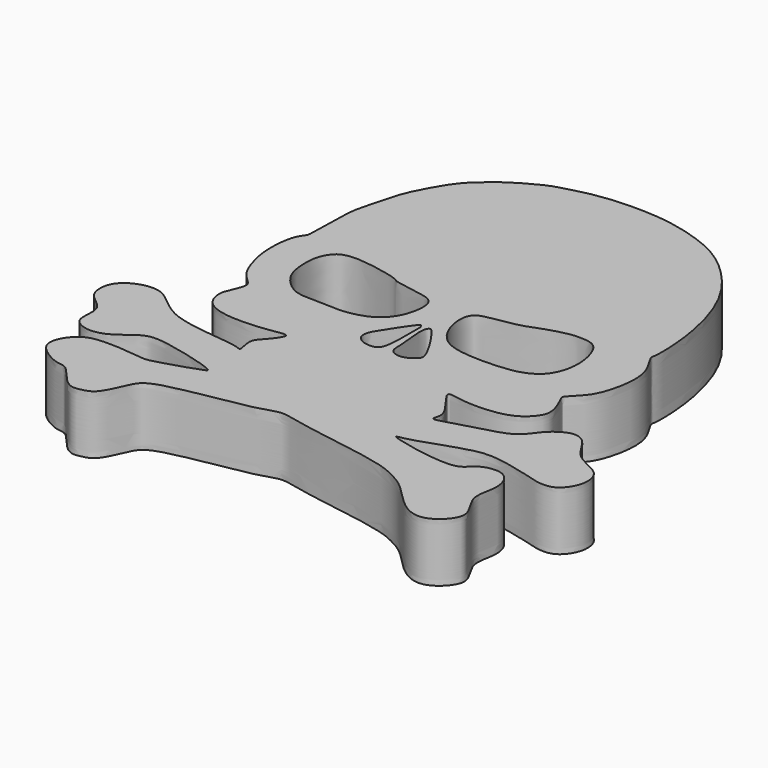
from build123d import *

# Parameters (mm, degrees)
F2_DEPTH = 5


# Not quite as in the source:
# - the program builds the solid bodies; features that only make, move or delete a surface that nothing else refers to are left out


with BuildPart() as f2:
    # F0 (on Top) → F2 (new body)
    with BuildSketch(Plane.XY):
        with BuildLine():
            add(Edge.make_bspline(
                [(0, 29.1948150843), (-0.455700376, 29.1905925458), (-1.1567215924, 29.1618461529), (-3.1403467697, 28.9760038822), (-5.3502695562, 28.3451092019), (-6.2987855508, 28.08405076), (-8.7371541954, 26.7472490664), (-9.9789020308, 25.6205862946), (-11.1795496875, 24.6292942159), (-12.7218376486, 21.8252572969), (-13.1883939862, 20.579718657), (-13.7634070057, 18.2333096853), (-14.1852851071, 16.8622027364), (-14.1170047877, 12.8287797099), (-14.2482133356, 12.4533380127), (-14.8390084605, 11.7676672429), (-15.0846571902, 9.4308819888), (-14.7559319963, 7.5205014424), (-14.0572172751, 5.5914730666), (-13.0121365975, 4.8260616544), (-12.7602375114, 4.229640466), (-13.3888684676, 2.9495519697), (-13.5820065327, 2.2406487992), (-13.2306782333, 0.8255751981), (-11.2533403548, -0.0175168629), (-7.8816952761, 0.2001522646), (-6.4944183105, 0.5344949605), (-6.1204957666, 0.2935652285), (-7.0327782743, -0.9471395034), (-7.8681534364, -1.650483246), (-7.2751479554, -3.2843527943), (-8.1628741959, -2.6478349983), (-13.7402125566, -2.5894083194), (-15.7791340083, -0.3730836673), (-17.1585341356, 0.3335309748), (-18.6083298281, 0.0772907355), (-19.5951663859, -0.5228293797), (-20.2156875042, -1.3707138004), (-20.2463078231, -3.2221635924), (-18.2278171957, -4.1070504005), (-18.5823469671, -5.9281770774), (-18.3237505227, -6.7522032766), (-17.1782189553, -7.2951260169), (-15.5290572679, -7.0027828669), (-13.8629059388, -5.4261850537), (-12.2189503414, -5.1810247155), (-6.8913491283, -6.5946613819), (-7.5377381272, -7.0092561754), (-11.2168759239, -8.1863406129), (-11.8490931224, -8.1033994548), (-16.1271497353, -7.5905806702), (-17.3629207849, -8.7236417952), (-17.9219651644, -9.6277084995), (-18.0488749277, -10.9819934587), (-16.0020742728, -12.1601073407), (-15.4317544768, -12.1457345363), (-14.7512786345, -12.3317850721), (-13.9026392621, -13.5370953675), (-12.8951873314, -14.3975838856), (-11.9433573754, -14.177352226), (-11.0274493069, -13.9390642999), (-10.2574160991, -12.2671019175), (-9.8684058522, -11.3195018224), (-8.8658318822, -10.1379170413), (-1.2058784185, -9.1883129388), (0.3235668746, -8.3151335086), (2.2820035826, -8.8832158896), (5.5927219878, -9.3985978575), (7.4139892784, -9.6776207077), (10.3878555066, -10.2681628014), (11.6014567723, -10.8226010538), (13.0999184497, -11.645353175), (14.5175313676, -13.3145860992), (16.0906457526, -14.4698757402), (17.5435543548, -14.4243517005), (18.8035028973, -13.3636768778), (19.3314294433, -11.9666989236), (17.5753238972, -10.0779106532), (18.5354487794, -7.8924152647), (17.5937222417, -5.7360265957), (15.0703828771, -6.234446849), (14.5648753095, -7.953261075), (7.5971964752, -6.4117846293), (9.442200865, -6.3071141647), (13.3764202735, -4.7285595175), (15.716513279, -4.4844330359), (19.4156937792, -5.5234901434), (19.861155828, -5.6546360397), (21.303419766, -5.8004753827), (22.300460868, -4.518839727), (22.5243431369, -3.3487826511), (22.0916128896, -1.9349896886), (19.6035203653, -1.2590429946), (18.8399693891, 0.765903237), (17.4346694984, 1.5410863929), (15.5716090748, 0.3176959724), (14.7747626125, -1.4624555319), (11.3649118248, -2.1276417927), (8.6284919308, -3.1306467762), (8.8522629011, -2.4946634527), (9.0670777263, -1.6343380568), (6.6516812, 0.8903161082), (8.6859227155, 0.3162393757), (11.0097092584, 0.3070352004), (13.019460402, 0.7530993219), (14.2545025425, 2.0366374807), (14.3418632854, 3.0634006451), (13.8345888548, 4.2908181196), (13.5602088632, 4.7609245882), (13.5445813704, 5.0931152788), (14.7192104011, 6.0611113985), (15.5243795175, 7.7812436707), (16.0362288926, 11.1198158729), (14.473678678, 12.9975581843), (14.749490572, 13.4709184724), (14.6206756183, 17.1320281508), (13.4949448137, 21.4665955495), (11.613169172, 24.5749660361), (8.8878900036, 27.1712648948), (6.0546332528, 28.3962254244), (2.9530896675, 29.173496563), (0.7107278145, 29.2014007177), (0, 29.1948150843)],
                knots=[0, 0, 0, 0, 0.0067947108, 0.0156804207, 0.0251148324, 0.0315587701, 0.0418748165, 0.0500983998, 0.0579736325, 0.0690221426, 0.0766762585, 0.0859780744, 0.0943425662, 0.1066479587, 0.1105575947, 0.1160757372, 0.1256064852, 0.1346582143, 0.1435568663, 0.1504675672, 0.1551760394, 0.162459216, 0.1680045462, 0.1749681561, 0.1838970634, 0.19570647, 0.2029492284, 0.2058819519, 0.2132033711, 0.220039621, 0.2269112182, 0.2313926808, 0.2461607994, 0.2571024927, 0.264545581, 0.2719544608, 0.2786172102, 0.2849261587, 0.2928512682, 0.3014803403, 0.3094344002, 0.3150245827, 0.3216554892, 0.3296807402, 0.3387684105, 0.3475915932, 0.3614746058, 0.3646340772, 0.3768443544, 0.383124006, 0.3956814227, 0.403623535, 0.4098863918, 0.416699982, 0.4259289189, 0.4307018278, 0.4356012085, 0.4432611025, 0.4503524484, 0.4562288853, 0.4621727355, 0.4705002364, 0.4767874895, 0.4842047659, 0.5015355296, 0.5100049396, 0.5185786191, 0.5300477109, 0.5390129764, 0.5497341771, 0.5570898483, 0.5651029201, 0.5745254162, 0.5831727936, 0.5903907555, 0.598246537, 0.6053638329, 0.614730315, 0.6241202322, 0.6327396515, 0.641575784, 0.6495582683, 0.6643914285, 0.6691930217, 0.682307442, 0.6928082846, 0.7046011432, 0.7091743205, 0.7161949635, 0.7239116167, 0.7307015612, 0.7377817415, 0.7474570773, 0.7564815119, 0.7637164238, 0.7725117749, 0.7809944805, 0.7929916457, 0.8027326768, 0.8061018421, 0.8121161908, 0.8221347891, 0.828597217, 0.8387005328, 0.8477238813, 0.8557102992, 0.8619500889, 0.8691617381, 0.8736916981, 0.8768297501, 0.8841376024, 0.8930523815, 0.9045534974, 0.9136542049, 0.917719434, 0.929301999, 0.9430324516, 0.9549843951, 0.9670043906, 0.9780032637, 0.9894027079, 1, 1, 1, 1], degree=3))
        make_face()
        with BuildLine():
            add(Edge.make_bspline(
                [(-0.256584317, 7.141367998), (-0.3160373469, 7.1538403671), (-0.4757799103, 6.9511854635), (-0.9549769091, 6.3068464939), (-1.6923599308, 5.1415561247), (-2.2969604587, 4.2584240453), (-2.4430958311, 3.4066857737), (-1.7904651594, 2.7195420637), (-0.4498707313, 2.6563231111), (-0.1046752505, 3.5124050288), (-0.0512294187, 5.1949870786), (-0.0815848313, 6.5344615874), (-0.0432850893, 6.8869453377), (-0.1913029283, 7.1276729251), (-0.256584317, 7.141367998)],
                knots=[0, 0, 0, 0, 0.0440834259, 0.1266881981, 0.2354788451, 0.3306498943, 0.4099057678, 0.4938051313, 0.5917524056, 0.6713757591, 0.7924579444, 0.8975645323, 0.9515949438, 1, 1, 1, 1], degree=3))
        make_face(mode=Mode.SUBTRACT)
        with BuildLine():
            add(Edge.make_bspline(
                [(0.5537052057, 7.0902686566), (0.4847157086, 7.065629918), (0.2462017696, 6.8272821787), (0.3505334284, 5.3409308334), (0.5402222252, 4.1345701722), (0.4455145051, 2.8994930838), (1.7407481462, 2.6394633793), (2.5275495977, 3.2551031165), (3.0670934574, 3.747499506), (0.899957098, 7.0037701506), (0.6208747848, 7.1142574343), (0.5537052057, 7.0902686566)],
                knots=[0, 0, 0, 0, 0.0606408934, 0.1916216523, 0.3195150268, 0.4303112671, 0.541942966, 0.6487175585, 0.729952521, 0.9409587914, 1, 1, 1, 1], degree=3))
        make_face(mode=Mode.SUBTRACT)
        with BuildLine():
            add(Edge.make_bspline(
                [(-9.4919735566, 11.9435777888), (-9.731856646, 11.9431339793), (-10.4025316241, 11.8985617041), (-11.1402226353, 11.585247135), (-11.6778499919, 10.6365273222), (-11.8387057244, 9.7543773642), (-11.8106747115, 8.2865570084), (-11.3769216794, 7.0120622529), (-10.2200794327, 5.8696790086), (-9.1228460064, 5.4778012806), (-7.3137774926, 5.512926788), (-5.5797910502, 5.3655267511), (-3.4325454861, 5.8702256548), (-2.3254590339, 7.008396917), (-1.8579200144, 8.1189424147), (-1.6438471983, 9.4466829035), (-2.0330106022, 10.471969184), (-3.5821192175, 10.6984959081), (-5.5618055504, 11.014339873), (-5.6055589145, 11.2734889759), (-7.7112442008, 11.7732942818), (-8.9920132873, 11.9123324613), (-9.3170524373, 11.9439014117), (-9.4919735566, 11.9435777888)],
                knots=[0, 0, 0, 0, 0.0401521642, 0.0782415524, 0.1212497591, 0.1621698062, 0.2132046853, 0.2631346044, 0.3161503068, 0.3618936274, 0.4184069205, 0.475986305, 0.5384398841, 0.5909998739, 0.6377570486, 0.6868022904, 0.7274317757, 0.7815450895, 0.8401644428, 0.8590453231, 0.920338809, 0.9707213146, 1, 1, 1, 1], degree=3))
        make_face(mode=Mode.SUBTRACT)
        with BuildLine():
            add(Edge.make_bspline(
                [(10.1495459676, 12.1967671439), (9.758199193, 12.3444542925), (8.9688719183, 12.3233603524), (8.7268898602, 12.3642856595), (6.8022443568, 12.0061540246), (4.7578706539, 11.0079932867), (2.0891989848, 10.8441071968), (1.2363093366, 10.1253259437), (1.2779229329, 8.5980810624), (1.8225051082, 7.1596266297), (3.078564706, 5.8701046484), (5.6837658037, 5.6352842722), (7.6366652334, 5.6999795852), (9.2942736505, 5.9143070841), (10.9282809854, 6.8381797704), (11.600424083, 9.1024585372), (11.1420008579, 11.2810889964), (10.5566235185, 12.0431434867), (10.1495459676, 12.1967671439)],
                knots=[0, 0, 0, 0, 0.0527108202, 0.0778999016, 0.1423217348, 0.2201304511, 0.2982159596, 0.3454305238, 0.4029753283, 0.4635398297, 0.5266762941, 0.6044288108, 0.6735209616, 0.7357213687, 0.7998797274, 0.8729478494, 0.9451703885, 1, 1, 1, 1], degree=3))
        make_face(mode=Mode.SUBTRACT)
    extrude(amount=F2_DEPTH)


solid = f2.part
